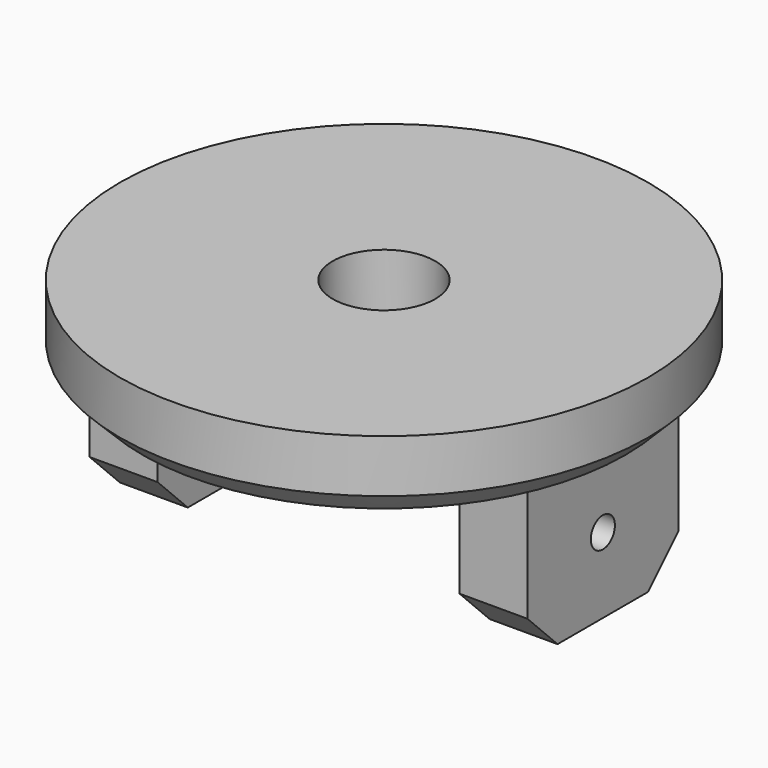
from build123d import *

# Parameters (mm, degrees)
F1_DEPTH  = 5
F3_SIZE   = 1
F2_W      = 4.5
F2_H      = 12.5
F4_DEPTH  = 10
F5_SIZE   = 2.5
F6_R      = 1
F7_DEPTH  = 39.5010001
F8_R      = 39.5864097355
F8_R_2    = 17.5
F9_DEPTH  = 25
F10_SIZE  = 1.5
F11_R     = 3.4
F12_DEPTH = 25


with BuildPart() as f1:
    # F0 (on Top) → F1 (new body)
    with BuildSketch(Plane.XY):
        with BuildLine():
            ThreePointArc((19.8625961196, -15.8301909188), (23.6080012184, -12.5093598908), (25, -7.7012087429))
            Line((25, -7.7012087429), (25, 7.7012087429))
            ThreePointArc((25, 7.7012087429), (23.6080012184, 12.5093598908), (19.8625961196, 15.8301909188))
            add(Edge.make_bspline(
                [(19.8625961196, 15.8301909188), (0, 25.2681728257), (-19.8625961196, 15.8301909188)],
                knots=[0.9132750433, 0.9132750433, 0.9132750433, 2.2283176103, 2.2283176103, 2.2283176103], degree=2, weights=[1, 0.7915095459, 1]))
            ThreePointArc((-19.8625961196, 15.8301909188), (-23.6080012184, 12.5093598908), (-25, 7.7012087429))
            Line((-25, 7.7012087429), (-25, -7.7012087429))
            ThreePointArc((-25, -7.7012087429), (-23.6080012184, -12.5093598908), (-19.8625961196, -15.8301909188))
            add(Edge.make_bspline(
                [(-19.8625961196, -15.8301909188), (0, -25.2681728257), (19.8625961196, -15.8301909188)],
                knots=[4.0548676969, 4.0548676969, 4.0548676969, 5.3699102639, 5.3699102639, 5.3699102639], degree=2, weights=[1, 0.7915095459, 1]))
        make_face()
    extrude(amount=F1_DEPTH)

    # F3
    f3_edges = [f1.edges().sort_by_distance(p)[0] for p in [
        (4e-06, -20, 0),
    ]]
    chamfer(f3_edges, length=F3_SIZE)

    # F2 (on face) → F4 (join)
    with BuildSketch(Plane(origin=(0, 0, 0), x_dir=(1, 0, 0), z_dir=(0, 0, -1))):
        with Locations((12.25, 0)):
            Rectangle(F2_W, F2_H)
        with Locations((-12.25, 0)):
            Rectangle(F2_W, F2_H)
    extrude(amount=F4_DEPTH)

    # F5
    f5_edges = [f1.edges().sort_by_distance(p)[0] for p in [
        (-12.25, -6.25, -10),
        (12.25, -6.25, -10),
        (-12.25, 6.25, -10),
        (12.25, 6.25, -10),
    ]]
    chamfer(f5_edges, length=F5_SIZE)

    # F6 (on face) → F7 (cut, through all)
    with BuildSketch(Plane.YZ.offset(14.5)):
        with Locations((0, -5)):
            Circle(F6_R)
    extrude(amount=-F7_DEPTH, mode=Mode.SUBTRACT)

    # F8 (on face) → F9 (cut)
    with BuildSketch(Plane.XY.offset(5)):
        Circle(F8_R)
        with BuildLine():
            add(Edge.make_bspline(
                [(-19.8625961196, -15.8301909188), (0, -25.2681728257), (19.8625961196, -15.8301909188)],
                knots=[4.0548676969, 4.0548676969, 4.0548676969, 5.3699102639, 5.3699102639, 5.3699102639], degree=2, weights=[1, 0.7915095459, 1]))
            ThreePointArc((-19.8625961196, -15.8301909188), (-23.6080012184, -12.5093598908), (-25, -7.7012087429))
            Line((-25, -7.7012087429), (-25, 7.7012087429))
            ThreePointArc((-25, 7.7012087429), (-23.6080012184, 12.5093598908), (-19.8625961196, 15.8301909188))
            add(Edge.make_bspline(
                [(19.8625961196, 15.8301909188), (0, 25.2681728257), (-19.8625961196, 15.8301909188)],
                knots=[0.9132750433, 0.9132750433, 0.9132750433, 2.2283176103, 2.2283176103, 2.2283176103], degree=2, weights=[1, 0.7915095459, 1]))
            ThreePointArc((19.8625961196, 15.8301909188), (23.6080012184, 12.5093598908), (25, 7.7012087429))
            Line((25, 7.7012087429), (25, -7.7012087429))
            ThreePointArc((25, -7.7012087429), (23.6080012184, -12.5093598908), (19.8625961196, -15.8301909188))
        make_face(mode=Mode.SUBTRACT)
        with BuildLine():
            ThreePointArc((-25, -7.7012087429), (-23.6080012184, -12.5093598908), (-19.8625961196, -15.8301909188))
            add(Edge.make_bspline(
                [(-19.8625961196, -15.8301909188), (0, -25.2681728257), (19.8625961196, -15.8301909188)],
                knots=[4.0548676969, 4.0548676969, 4.0548676969, 5.3699102639, 5.3699102639, 5.3699102639], degree=2, weights=[1, 0.7915095459, 1]))
            ThreePointArc((19.8625961196, -15.8301909188), (23.6080012184, -12.5093598908), (25, -7.7012087429))
            Line((25, -7.7012087429), (25, 7.7012087429))
            ThreePointArc((25, 7.7012087429), (23.6080012184, 12.5093598908), (19.8625961196, 15.8301909188))
            add(Edge.make_bspline(
                [(19.8625961196, 15.8301909188), (0, 25.2681728257), (-19.8625961196, 15.8301909188)],
                knots=[0.9132750433, 0.9132750433, 0.9132750433, 2.2283176103, 2.2283176103, 2.2283176103], degree=2, weights=[1, 0.7915095459, 1]))
            ThreePointArc((-19.8625961196, 15.8301909188), (-23.6080012184, 12.5093598908), (-25, 7.7012087429))
            Line((-25, 7.7012087429), (-25, -7.7012087429))
        make_face()
        Circle(F8_R_2, mode=Mode.SUBTRACT)
    extrude(amount=-F9_DEPTH, mode=Mode.SUBTRACT)

    # F10
    f10_edges = [f1.edges().sort_by_distance(p)[0] for p in [
        (-17.5, 0, 0),
    ]]
    chamfer(f10_edges, length=F10_SIZE)

    # F11 (on face) → F12 (cut)
    with BuildSketch(Plane.XY.offset(5)):
        Circle(F11_R)
    extrude(amount=-F12_DEPTH, mode=Mode.SUBTRACT)


solid = f1.part
